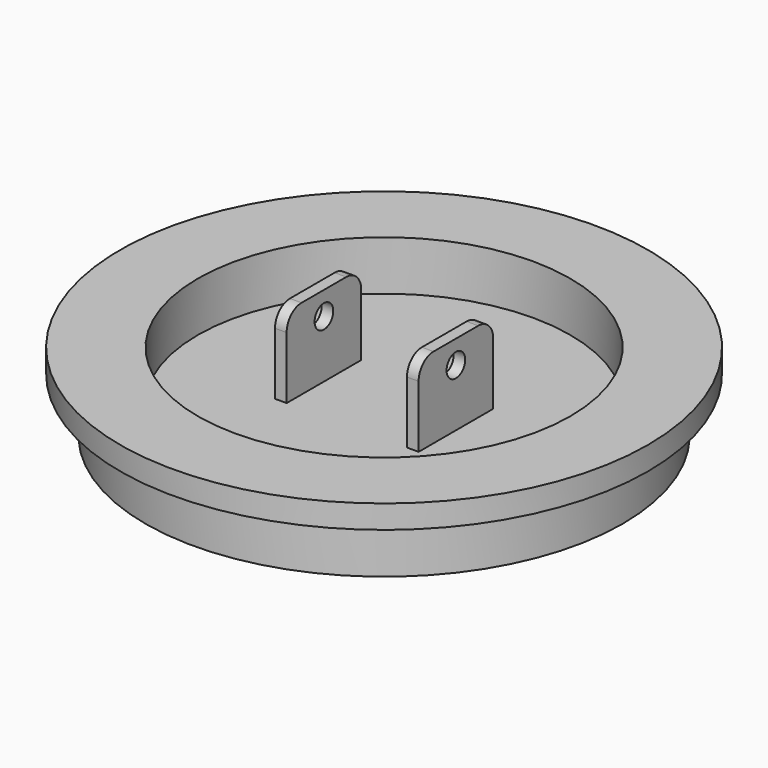
from build123d import *

# Parameters (mm, degrees)
F0_R      = 16.271875
F0_R_2    = 12.7
F1_DEPTH  = 5.2916666667
F2_START  = 3.7041666667
F0_R_3    = 17.9916666667
F2_DEPTH  = 1.5875
F3_R      = 13.97
F4_DEPTH  = 1.905
F5_DEPTH  = 1.27
F6_W      = 0.79375
F6_H      = 6.35
F7_DEPTH  = 7.4083333333
F8_R      = 1.27
F9_R      = 0.79375
F10_DEPTH = 25.4


with BuildPart() as f1:
    # F0 (on Top) → F1 (new body)
    with BuildSketch(Plane.XY):
        Circle(F0_R)
        Circle(F0_R_2, mode=Mode.SUBTRACT)
    extrude(amount=F1_DEPTH)

    # F0 (on Top) → F2 (join)
    with BuildSketch(Plane.XY.offset(F2_START)):
        Circle(F0_R_3)
        Circle(F0_R, mode=Mode.SUBTRACT)
    extrude(amount=F2_DEPTH)

    # F3 (on Top) → F5 (cut)
    with BuildSketch(Plane.XY):
        Circle(F3_R)
    extrude(amount=F5_DEPTH, mode=Mode.SUBTRACT)


with BuildPart() as f4:
    # F3 (on Top) → F4 (new body)
    with BuildSketch(Plane.XY):
        Circle(F3_R)
    extrude(amount=F4_DEPTH)

    # F6 (on Top) → F7 (join)
    with BuildSketch(Plane.XY):
        with Locations((-4.4979166667, 0)):
            Rectangle(F6_W, F6_H)
        with Locations((4.4979166667, 0)):
            Rectangle(F6_W, F6_H)
    extrude(amount=F7_DEPTH)

    # F8
    f8_edges = [f4.edges().sort_by_distance(p)[0] for p in [
        (-4.497917, -3.175, 7.408333),
        (4.497917, -3.175, 7.408333),
        (4.497917, 3.175, 7.408333),
        (-4.497917, 3.175, 7.408333),
    ]]
    fillet(f8_edges, radius=F8_R)

    # F9 (on face) → F10 (cut)
    with BuildSketch(Plane(origin=(-4.8947916667, 0, 0), x_dir=(0, -1, 0), z_dir=(-1, 0, 0))):
        with Locations((0, 5.8208333333)):
            Circle(F9_R)
    extrude(amount=-F10_DEPTH, mode=Mode.SUBTRACT)


solid = Compound([f1.part, f4.part])
